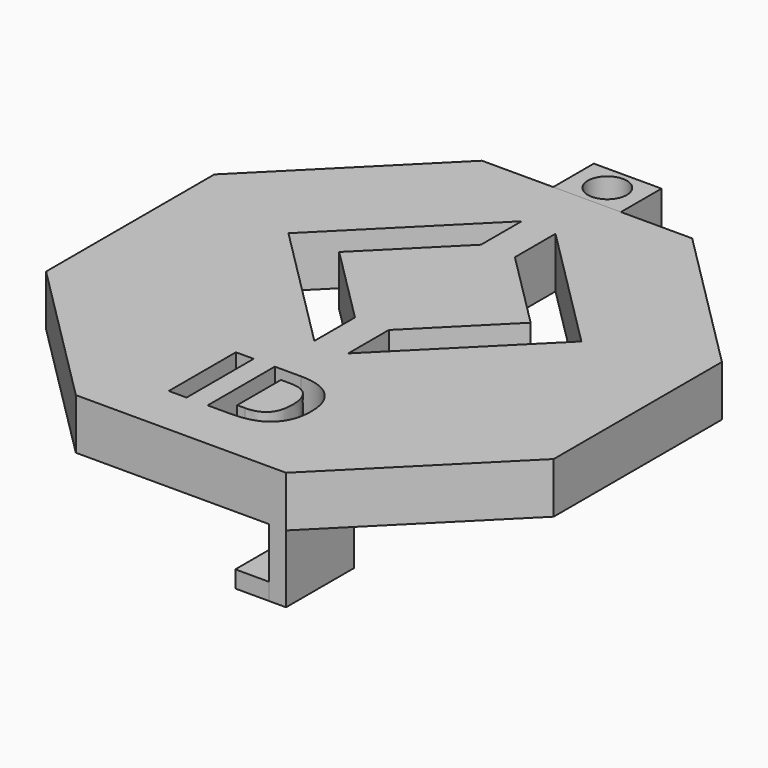
from build123d import *

# Parameters (mm, degrees)
F1_DEPTH     = 3
F2_TEXT_SIZE = 6.9444444444
F3_DEPTH     = 3.001
F4_W         = 1
F4_H         = 5
F5_DEPTH     = 4
F6_W         = 5
F6_H         = 1
F7_DEPTH     = 2
F8_W         = 4
F8_H         = 3
F9_DEPTH     = 3
F10_R        = 1.15
F11_DEPTH    = 3.0010001


# Not quite as in the source:
# - Text() gives the source's letters only with a copy of the font that has no kerning and outlines rounded to 1/6400 em; it was checked with that copy


with BuildPart() as f1:
    # F0 (on Top) → F1 (new body)
    with BuildSketch(Plane.XY):
        Polygon((15, -6.2132034356), (15, 6.2132034356), (6.2132034356, 15), (-6.2132034356, 15), (-15, 6.2132034356), (-15, -6.2132034356), (-6.2132034356, -15), (6.2132034356, -15), align=None)
    extrude(amount=F1_DEPTH)

    # F2 (on face) → F3 (cut, through all)
    with BuildSketch(Plane.XY.offset(3)):
        Polygon((1, 8.418436326), (5.6568542495, 3.7615820765), (1, -0.8952721729), (1, -3.8952721729), (8.6568542495, 3.7615820765), (1, 11.418436326), align=None)
        Polygon((-1, -0.8952721729), (-5.6568542495, 3.7615820765), (-1, 8.418436326), (-1, 11.418436326), (-8.6568542495, 3.7615820765), (-1, -3.8952721729), align=None)
        with Locations((-3.7434895833, -12)):
            Text('ID', F2_TEXT_SIZE, font='Open Sans', font_style=FontStyle.BOLD, text_align=(TextAlign.LEFT, TextAlign.BOTTOM))
    extrude(amount=-F3_DEPTH, mode=Mode.SUBTRACT)

    # F4 (on face) → F5 (join)
    with BuildSketch(Plane(origin=(0, 0, 0), x_dir=(1, 0, 0), z_dir=(0, 0, -1))):
        with Locations((5.7132034356, 12.5)):
            Rectangle(F4_W, F4_H)
    extrude(amount=F5_DEPTH)


with BuildPart() as f7:
    # F6 (on face) → F7 (new body)
    with BuildSketch(Plane(origin=(5.2132034356, 0, 0), x_dir=(0, -1, 0), z_dir=(-1, 0, 0))):
        with Locations((12.5, -3.5)):
            Rectangle(F6_W, F6_H)
    extrude(amount=F7_DEPTH)


with BuildPart() as f9:
    # F8 (on face) → F9 (new body)
    with BuildSketch(Plane(origin=(0, 15, 0), x_dir=(-1, 0, 0), z_dir=(0, 1, 0))):
        with Locations((0, 1.5)):
            Rectangle(F8_W, F8_H)
    extrude(amount=F9_DEPTH)

    # F10 (on face) → F11 (cut, through all)
    with BuildSketch(Plane(origin=(0, 0, 0), x_dir=(1, 0, 0), z_dir=(0, 0, -1))):
        with Locations((0, -16.5)):
            Circle(F10_R)
    extrude(amount=-F11_DEPTH, mode=Mode.SUBTRACT)


solid = Compound([f1.part, f7.part, f9.part])
